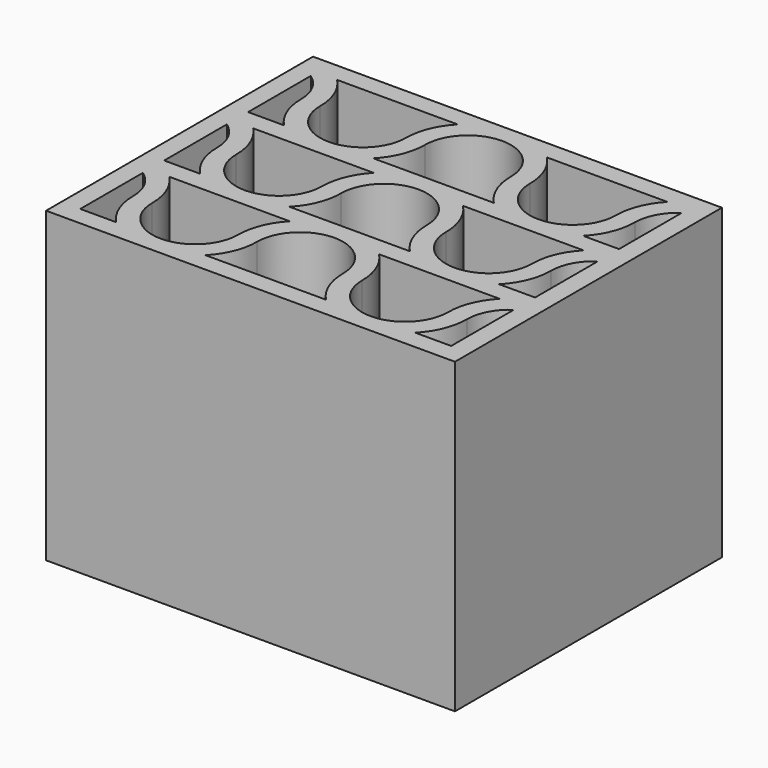
from build123d import *

# Parameters (mm, degrees)
F0_W     = 107.602417469
F0_H     = 87.8107035317
F1_DEPTH = 81


# Not quite as in the source:
# - ends of sketch curves that miss each other by under 0.0002 mm in the source are joined


with BuildPart() as f1:
    # F0 (on Top) → F1 (new body)
    with BuildSketch(Plane.XY):
        Rectangle(F0_W, F0_H)
        with BuildLine():
            Line((-43.4592129171, -38.9053517658), (-48.8012087345, -38.9053517658))
            Line((-48.8012087345, -38.9053517658), (-48.8012087345, -18.2926106175))
            ThreePointArc((-48.8012087345, -18.2926106175), (-45.2040241526, -22.3437425741), (-43.9055000032, -27.6035184325))
            ThreePointArc((-43.9055000032, -27.6035184325), (-42.8947395838, -33.2544350992), (-39.987798415, -38.2046056862))
            ThreePointArc((-39.987798415, -38.2046056862), (-39.6614460497, -38.566308994), (-39.3116101623, -38.9053517658))
            Line((-39.3116101623, -38.9053517658), (-43.4592129171, -38.9053517658))
        make_face(mode=Mode.SUBTRACT)
        with BuildLine():
            ThreePointArc((-38.9055000032, -27.6035184325), (-40.0867237079, -21.511151528), (-43.4592129171, -16.3016850991))
            Line((-43.4592129171, -16.3016850991), (-11.748120417, -16.3016850991))
            ThreePointArc((-11.748120417, -16.3016850991), (-15.120609628, -21.5111515275), (-16.3018333334, -27.6035184325))
            ThreePointArc((-16.3018333334, -27.6035184325), (-27.6036666683, -38.9053517674), (-38.9055000032, -27.6035184325))
        make_face(mode=Mode.SUBTRACT)
        with BuildLine():
            Line((-43.4586830682, -11.3016850991), (-48.8012087345, -11.3016850991))
            Line((-48.8012087345, -11.3016850991), (-48.8012087345, 9.3111358172))
            ThreePointArc((-48.8012087345, 9.3111358172), (-45.2037061615, 5.2599802444), (-43.9050552974, 0))
            ThreePointArc((-43.9050552974, 0), (-42.7238541219, -6.0922822479), (-39.3514275267, -11.3016850991))
            Line((-39.3514275267, -11.3016850991), (-43.4586830682, -11.3016850991))
        make_face(mode=Mode.SUBTRACT)
        with BuildLine():
            ThreePointArc((-11.3018333334, -27.6035184325), (0, -16.3016850991), (11.3018333333, -27.6035184325))
            ThreePointArc((11.3018333334, -27.6035184325), (12.4830570387, -33.6958853375), (15.8555462497, -38.9053517658))
            Line((15.8555462497, -38.9053517658), (-15.8555462474, -38.9053517658))
            ThreePointArc((-15.8555462474, -38.9053517658), (-12.4830570378, -33.6958853372), (-11.3018333334, -27.6035184325))
        make_face(mode=Mode.SUBTRACT)
        with BuildLine():
            ThreePointArc((38.9055, -27.6035184325), (27.6036666667, -38.9053517658), (16.3018333334, -27.6035184325))
            ThreePointArc((16.3018333334, -27.6035184325), (15.120609628, -21.5111515275), (11.748120417, -16.3016850991))
            Line((11.748120417, -16.3016850991), (43.4592129164, -16.3016850991))
            ThreePointArc((43.4592129164, -16.3016850991), (40.0867237054, -21.5111515275), (38.9055, -27.6035184325))
        make_face(mode=Mode.SUBTRACT)
        with BuildLine():
            ThreePointArc((43.9055, -27.6035184325), (45.2040241503, -22.3437425739), (48.8012087345, -18.2926106186))
            Line((48.8012087345, -18.2926106186), (48.8012087345, -38.9053517658))
            Line((48.8012087345, -38.9053517658), (43.4592129164, -38.9053517658))
            Line((43.4592129164, -38.9053517658), (39.3517870837, -38.9053517658))
            ThreePointArc((39.3517870837, -38.9053517658), (42.7242762947, -33.6958853375), (43.9055, -27.6035184325))
        make_face(mode=Mode.SUBTRACT)
        with BuildLine():
            Line((15.855319758, 11.3016850991), (43.4586830625, 11.3016850991))
            ThreePointArc((43.4586830625, 11.3016850991), (40.0862564691, 6.0922822475), (38.9050552942, 0))
            ThreePointArc((38.9050553006, 0), (27.6033701999, -11.3016851007), (16.3016850991, 0))
            ThreePointArc((16.3016850991, 0), (15.1204839236, 6.0922822479), (11.7480573284, 11.3016850991))
            Line((11.7480573284, 11.3016850991), (15.855319758, 11.3016850991))
        make_face(mode=Mode.SUBTRACT)
        with BuildLine():
            ThreePointArc((43.9050552942, 0), (45.2037061591, 5.2599802476), (48.8012087345, 9.3111358227))
            Line((48.8012087345, 9.3111358227), (48.8012087345, -11.3016850991))
            Line((48.8012087345, -11.3016850991), (43.4586830625, -11.3016850991))
            Line((43.4586830625, -11.3016850991), (39.3514275289, -11.3016850991))
            ThreePointArc((39.3514275289, -11.3016850991), (42.7238548196, -6.0922824277), (43.9050552942, 0))
        make_face(mode=Mode.SUBTRACT)
        with BuildLine():
            ThreePointArc((-16.3016850991, 0), (-27.6033701983, -11.3016850991), (-38.9050552974, 0))
            ThreePointArc((-38.9050552974, 0), (-40.086256473, 6.0922822479), (-43.4586830682, 11.3016850991))
            Line((-43.4586830682, 11.3016850991), (-15.8553128699, 11.3016850991))
            Line((-15.8553128699, 11.3016850991), (-11.7480573284, 11.3016850991))
            ThreePointArc((-11.7480573284, 11.3016850991), (-15.1204839236, 6.0922822479), (-16.3016850991, 0))
        make_face(mode=Mode.SUBTRACT)
        with BuildLine():
            Line((-48.8012087345, 16.3016850991), (-48.8012087345, 36.9144262464))
            ThreePointArc((-48.8012087345, 36.9144262464), (-45.2040241503, 32.8632942911), (-43.9055, 27.6035184325))
            ThreePointArc((-43.9055, 27.6035184325), (-42.7242762947, 21.5111515275), (-39.3517870837, 16.3016850991))
            Line((-39.3517870837, 16.3016850991), (-43.4592129164, 16.3016850991))
            Line((-43.4592129164, 16.3016850991), (-48.8012087345, 16.3016850991))
        make_face(mode=Mode.SUBTRACT)
        with BuildLine():
            ThreePointArc((-38.9055, 27.6035184325), (-40.0867237054, 33.6958853375), (-43.4592129164, 38.9053517658))
            Line((-43.4592129164, 38.9053517658), (-15.8555462497, 38.9053517658))
            Line((-15.8555462497, 38.9053517658), (-11.748120417, 38.9053517658))
            ThreePointArc((-11.748120417, 38.9053517658), (-15.120609628, 33.6958853375), (-16.3018333334, 27.6035184325))
            ThreePointArc((-16.3018333334, 27.6035184325), (-27.6036666667, 16.3016850991), (-38.9055, 27.6035184325))
        make_face(mode=Mode.SUBTRACT)
        with BuildLine():
            ThreePointArc((-11.3016850991, 0), (0, 11.3016850991), (11.3016850991, 0))
            ThreePointArc((11.3016850991, 0), (12.4805105623, -6.0863826289), (15.8464978932, -11.2925148079))
            ThreePointArc((15.8464978932, -11.2925148079), (15.8510483075, -11.2971849132), (15.8557668328, -11.3016850991))
            Line((15.8557668328, -11.3016850991), (-15.8553128699, -11.3016850991))
            ThreePointArc((-15.8553128699, -11.3016850991), (-12.4828862747, -6.0922822479), (-11.3016850991, 0))
        make_face(mode=Mode.SUBTRACT)
        with BuildLine():
            ThreePointArc((-11.3018333334, 27.6035184325), (0, 38.9053517658), (11.3018333334, 27.6035184325))
            ThreePointArc((11.3018333334, 27.6035184325), (12.4806822619, 21.5170487891), (15.8467347518, 16.310851698))
            ThreePointArc((15.8467347518, 16.310851698), (15.8512041563, 16.3060464442), (15.8561076969, 16.3016850991))
            Line((15.8561076969, 16.3016850991), (-15.8555462497, 16.3016850991))
            ThreePointArc((-15.8555462497, 16.3016850991), (-12.4830570387, 21.5111515275), (-11.3018333334, 27.6035184325))
        make_face(mode=Mode.SUBTRACT)
        with BuildLine():
            ThreePointArc((38.9055, 27.6035184325), (27.6036666667, 16.3016850991), (16.3018333334, 27.6035184325))
            ThreePointArc((16.3018333334, 27.6035184325), (15.120609628, 33.6958853375), (11.748120417, 38.9053517658))
            Line((11.748120417, 38.9053517658), (15.8555462497, 38.9053517658))
            Line((15.8555462497, 38.9053517658), (43.4592129164, 38.9053517658))
            ThreePointArc((43.4592129164, 38.9053517658), (40.0867237054, 33.6958853375), (38.9055, 27.6035184325))
        make_face(mode=Mode.SUBTRACT)
        with BuildLine():
            ThreePointArc((43.9055, 27.6035184325), (45.2040241503, 32.8632942911), (48.8012087345, 36.9144262464))
            Line((48.8012087345, 36.9144262464), (48.8012087345, 27.6035184325))
            Line((48.8012087345, 27.6035184325), (48.8012087345, 16.3016850991))
            Line((48.8012087345, 16.3016850991), (43.4592129164, 16.3016850991))
            Line((43.4592129164, 16.3016850991), (39.3517870837, 16.3016850991))
            ThreePointArc((39.3517870837, 16.3016850991), (42.7242762947, 21.5111515275), (43.9055, 27.6035184325))
        make_face(mode=Mode.SUBTRACT)
    extrude(amount=F1_DEPTH)


solid = f1.part
